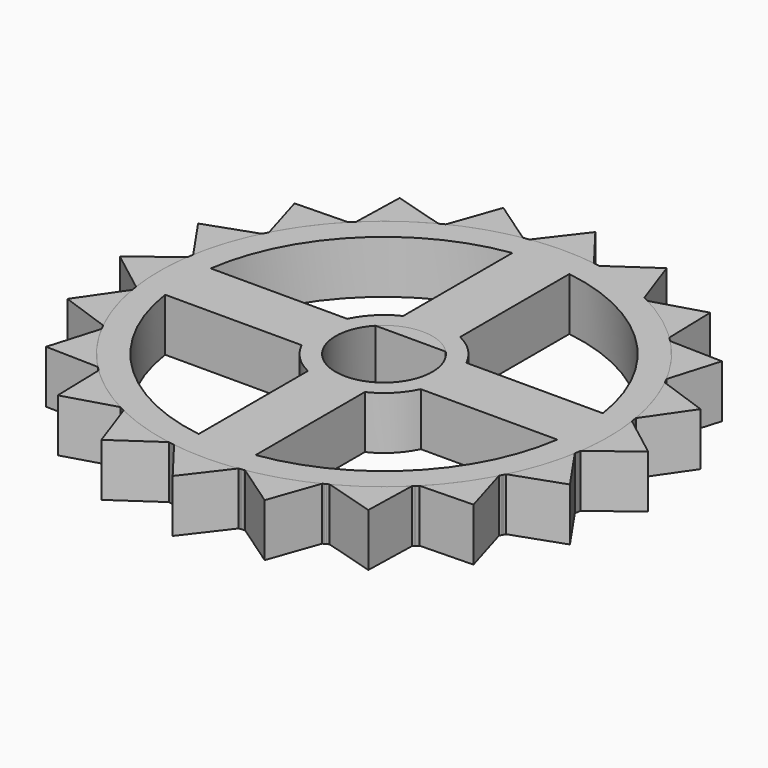
from build123d import *

# Parameters (mm, degrees)
F1_DEPTH = 6
F3_COUNT = 20
F4_DEPTH = 6
F6_DEPTH = 6


with BuildPart() as f1:
    # F0 (on Top) → F1 (new body)
    with BuildSketch(Plane.XY):
        with BuildLine():
            ThreePointArc((-3.649464858, 25.2375), (-16.6911450494, -19.278373296), (25.5, 0))
            ThreePointArc((25.5, 0), (19.278373296, 16.6911450494), (3.649464858, 25.2375))
            ThreePointArc((3.649464858, 25.2375), (0, 25.5), (-3.649464858, 25.2375))
        make_face()
        with BuildLine():
            ThreePointArc((4, 3.7749172176), (5.1112620751, 2.0310096012), (5.5, 0))
            ThreePointArc((5.5, 0), (-2.0310096012, -5.1112620751), (-4, 3.7749172176))
            ThreePointArc((-4, 3.7749172176), (0, 5.5), (4, 3.7749172176))
        make_face(mode=Mode.SUBTRACT)
        with BuildLine():
            ThreePointArc((-3.649464858, 25.2375), (0, 25.5), (3.649464858, 25.2375))
            Line((3.649464858, 25.2375), (0, 30))
            Line((0, 30), (-3.649464858, 25.2375))
        make_face()
    extrude(amount=F1_DEPTH)


with BuildPart() as f3_1:
    # F3: instance of F1
    add(f1.part.rotate(Axis((0, 0, 9.4146067277), (0, 0, 1)), 1 * 360 / F3_COUNT))


with BuildPart() as f3_2:
    # F3: instance of F1
    add(f1.part.rotate(Axis((0, 0, 9.4146067277), (0, 0, 1)), 2 * 360 / F3_COUNT))


with BuildPart() as f3_3:
    # F3: instance of F1
    add(f1.part.rotate(Axis((0, 0, 9.4146067277), (0, 0, 1)), 3 * 360 / F3_COUNT))


with BuildPart() as f3_4:
    # F3: instance of F1
    add(f1.part.rotate(Axis((0, 0, 9.4146067277), (0, 0, 1)), 4 * 360 / F3_COUNT))


with BuildPart() as f3_5:
    # F3: instance of F1
    add(f1.part.rotate(Axis((0, 0, 9.4146067277), (0, 0, 1)), 5 * 360 / F3_COUNT))


with BuildPart() as f3_6:
    # F3: instance of F1
    add(f1.part.rotate(Axis((0, 0, 9.4146067277), (0, 0, 1)), 6 * 360 / F3_COUNT))


with BuildPart() as f3_7:
    # F3: instance of F1
    add(f1.part.rotate(Axis((0, 0, 9.4146067277), (0, 0, 1)), 7 * 360 / F3_COUNT))


with BuildPart() as f3_8:
    # F3: instance of F1
    add(f1.part.rotate(Axis((0, 0, 9.4146067277), (0, 0, 1)), 8 * 360 / F3_COUNT))


with BuildPart() as f3_9:
    # F3: instance of F1
    add(f1.part.rotate(Axis((0, 0, 9.4146067277), (0, 0, 1)), 9 * 360 / F3_COUNT))


with BuildPart() as f3_10:
    # F3: instance of F1
    add(f1.part.rotate(Axis((0, 0, 9.4146067277), (0, 0, 1)), 10 * 360 / F3_COUNT))


with BuildPart() as f3_11:
    # F3: instance of F1
    add(f1.part.rotate(Axis((0, 0, 9.4146067277), (0, 0, 1)), 11 * 360 / F3_COUNT))


with BuildPart() as f3_12:
    # F3: instance of F1
    add(f1.part.rotate(Axis((0, 0, 9.4146067277), (0, 0, 1)), 12 * 360 / F3_COUNT))


with BuildPart() as f3_13:
    # F3: instance of F1
    add(f1.part.rotate(Axis((0, 0, 9.4146067277), (0, 0, 1)), 13 * 360 / F3_COUNT))


with BuildPart() as f3_14:
    # F3: instance of F1
    add(f1.part.rotate(Axis((0, 0, 9.4146067277), (0, 0, 1)), 14 * 360 / F3_COUNT))


with BuildPart() as f3_15:
    # F3: instance of F1
    add(f1.part.rotate(Axis((0, 0, 9.4146067277), (0, 0, 1)), 15 * 360 / F3_COUNT))


with BuildPart() as f3_16:
    # F3: instance of F1
    add(f1.part.rotate(Axis((0, 0, 9.4146067277), (0, 0, 1)), 16 * 360 / F3_COUNT))


with BuildPart() as f3_17:
    # F3: instance of F1
    add(f1.part.rotate(Axis((0, 0, 9.4146067277), (0, 0, 1)), 17 * 360 / F3_COUNT))


with BuildPart() as f3_18:
    # F3: instance of F1
    add(f1.part.rotate(Axis((0, 0, 9.4146067277), (0, 0, 1)), 18 * 360 / F3_COUNT))


with BuildPart() as f3_19:
    # F3: instance of F1
    add(f1.part.rotate(Axis((0, 0, 9.4146067277), (0, 0, 1)), 19 * 360 / F3_COUNT))


with BuildPart() as f4:
    # F0 (on Top) → F4 (new body)
    with BuildSketch(Plane.XY):
        with BuildLine():
            Line((-4, 3.7749172176), (4, 3.7749172176))
            ThreePointArc((4, 3.7749172176), (0, 5.5), (-4, 3.7749172176))
        make_face()
    extrude(amount=F4_DEPTH)


with BuildPart() as f6_tool:
    # F5 (on face) → F6 (new body)
    with BuildSketch(Plane.XY.offset(6)):
        with BuildLine():
            ThreePointArc((3.2356603528, 6.7661290323), (5.3033008589, 5.3033008589), (6.7661290323, 3.2356603528))
            Line((6.7661290323, 3.2356603528), (22.2661290323, 3.2356603528))
            ThreePointArc((22.2661290323, 3.2356603528), (15.9099025767, 15.9099025767), (3.2356603528, 22.2661290323))
            Line((3.2356603528, 22.2661290323), (3.2356603528, 6.7661290323))
        make_face()
        with BuildLine():
            Line((-3.2356603528, -22.2661290323), (-3.2356603528, -6.7661290323))
            ThreePointArc((-3.2356603528, -6.7661290323), (-5.3033008589, -5.3033008589), (-6.7661290323, -3.2356603528))
            Line((-6.7661290323, -3.2356603528), (-22.2661290323, -3.2356603528))
            ThreePointArc((-22.2661290323, -3.2356603528), (-15.9099025767, -15.9099025767), (-3.2356603528, -22.2661290323))
        make_face()
        with BuildLine():
            Line((22.2661290323, -3.2356603528), (6.7661290323, -3.2356603528))
            ThreePointArc((6.7661290323, -3.2356603528), (5.3033008589, -5.3033008589), (3.2356603528, -6.7661290323))
            Line((3.2356603528, -6.7661290323), (3.2356603528, -22.2661290323))
            ThreePointArc((3.2356603528, -22.2661290323), (15.9099025767, -15.9099025767), (22.2661290323, -3.2356603528))
        make_face()
        with BuildLine():
            ThreePointArc((-6.7661290323, 3.2356603528), (-5.3033008589, 5.3033008589), (-3.2356603528, 6.7661290323))
            Line((-3.2356603528, 6.7661290323), (-3.2356603528, 22.2661290323))
            ThreePointArc((-3.2356603528, 22.2661290323), (-15.9099025767, 15.9099025767), (-22.2661290323, 3.2356603528))
            Line((-22.2661290323, 3.2356603528), (-6.7661290323, 3.2356603528))
        make_face()
    extrude(amount=-F6_DEPTH)


with BuildPart() as f1_1:
    add(f1.part)

    # F6: cut by f6_tool
    add(f6_tool.part, mode=Mode.SUBTRACT)


with BuildPart() as f3_1_1:
    add(f3_1.part)

    # F6: cut by f6_tool
    add(f6_tool.part, mode=Mode.SUBTRACT)


with BuildPart() as f3_2_1:
    add(f3_2.part)

    # F6: cut by f6_tool
    add(f6_tool.part, mode=Mode.SUBTRACT)


with BuildPart() as f3_3_1:
    add(f3_3.part)

    # F6: cut by f6_tool
    add(f6_tool.part, mode=Mode.SUBTRACT)


with BuildPart() as f3_4_1:
    add(f3_4.part)

    # F6: cut by f6_tool
    add(f6_tool.part, mode=Mode.SUBTRACT)


with BuildPart() as f3_5_1:
    add(f3_5.part)

    # F6: cut by f6_tool
    add(f6_tool.part, mode=Mode.SUBTRACT)


with BuildPart() as f3_6_1:
    add(f3_6.part)

    # F6: cut by f6_tool
    add(f6_tool.part, mode=Mode.SUBTRACT)


with BuildPart() as f3_7_1:
    add(f3_7.part)

    # F6: cut by f6_tool
    add(f6_tool.part, mode=Mode.SUBTRACT)


with BuildPart() as f3_8_1:
    add(f3_8.part)

    # F6: cut by f6_tool
    add(f6_tool.part, mode=Mode.SUBTRACT)


with BuildPart() as f3_9_1:
    add(f3_9.part)

    # F6: cut by f6_tool
    add(f6_tool.part, mode=Mode.SUBTRACT)


with BuildPart() as f3_10_1:
    add(f3_10.part)

    # F6: cut by f6_tool
    add(f6_tool.part, mode=Mode.SUBTRACT)


with BuildPart() as f3_11_1:
    add(f3_11.part)

    # F6: cut by f6_tool
    add(f6_tool.part, mode=Mode.SUBTRACT)


with BuildPart() as f3_12_1:
    add(f3_12.part)

    # F6: cut by f6_tool
    add(f6_tool.part, mode=Mode.SUBTRACT)


with BuildPart() as f3_13_1:
    add(f3_13.part)

    # F6: cut by f6_tool
    add(f6_tool.part, mode=Mode.SUBTRACT)


with BuildPart() as f3_14_1:
    add(f3_14.part)

    # F6: cut by f6_tool
    add(f6_tool.part, mode=Mode.SUBTRACT)


with BuildPart() as f3_15_1:
    add(f3_15.part)

    # F6: cut by f6_tool
    add(f6_tool.part, mode=Mode.SUBTRACT)


with BuildPart() as f3_16_1:
    add(f3_16.part)

    # F6: cut by f6_tool
    add(f6_tool.part, mode=Mode.SUBTRACT)


with BuildPart() as f3_17_1:
    add(f3_17.part)

    # F6: cut by f6_tool
    add(f6_tool.part, mode=Mode.SUBTRACT)


with BuildPart() as f3_18_1:
    add(f3_18.part)

    # F6: cut by f6_tool
    add(f6_tool.part, mode=Mode.SUBTRACT)


with BuildPart() as f3_19_1:
    add(f3_19.part)

    # F6: cut by f6_tool
    add(f6_tool.part, mode=Mode.SUBTRACT)


solid = Compound([f4.part, f1_1.part, f3_1_1.part, f3_2_1.part, f3_3_1.part, f3_4_1.part, f3_5_1.part, f3_6_1.part, f3_7_1.part, f3_8_1.part, f3_9_1.part, f3_10_1.part, f3_11_1.part, f3_12_1.part, f3_13_1.part, f3_14_1.part, f3_15_1.part, f3_16_1.part, f3_17_1.part, f3_18_1.part, f3_19_1.part])
